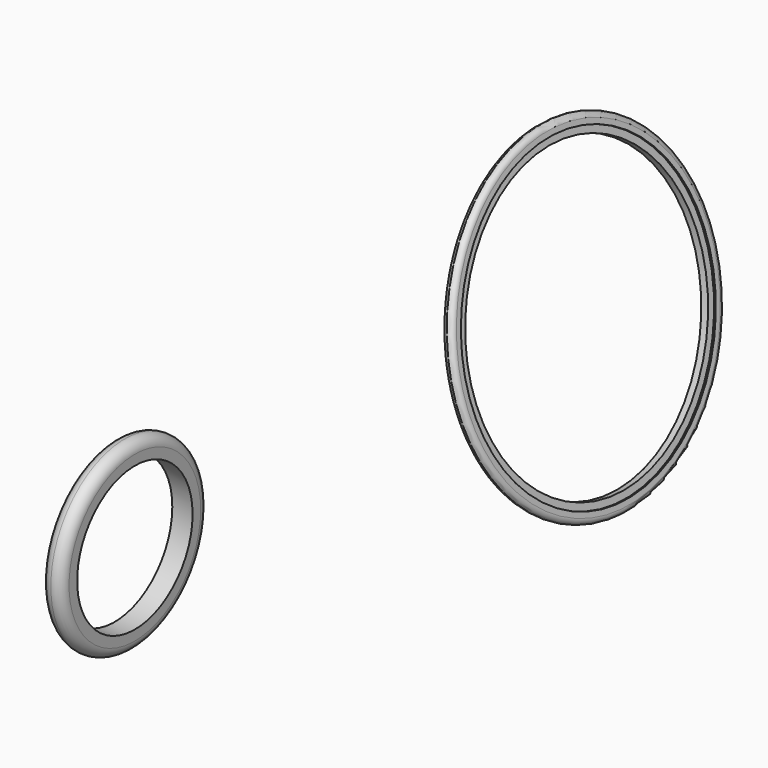
from build123d import *

# Parameters (mm, degrees)
F10_R     = 260.35
F10_R_2   = 203.2
F11_DEPTH = 28.575
F12_R     = 28.57499
F14_R     = 457.2
F14_R_2   = 427.2
F15_DEPTH = 15
F16_R     = 14.99999
F17_R     = 427.2
F17_R_2   = 407.2
F18_DEPTH = 10


# Not quite as in the source:
# - a fillet or chamfer is up to 0.001 mm smaller than in the source, because OpenCascade refuses the exact size


with BuildPart() as f11:
    # F10 (on Right) → F11 (new body, symmetric)
    with BuildSketch(Plane.YZ):
        with Locations((-600, 260.35)):
            Circle(F10_R)
        with Locations((-600, 260.35)):
            Circle(F10_R_2, mode=Mode.SUBTRACT)
    extrude(amount=F11_DEPTH, both=True)

    # F12 (radius 28.575 in the source; OpenCascade refuses exactly that, so slightly less here)
    f12_edges = [f11.edges().sort_by_distance(p)[0] for p in [
        (-28.575, -860.35, 260.35),
        (0, -339.65, 260.35),
        (28.575, -860.35, 260.35),
    ]]
    fillet(f12_edges, radius=F12_R)


with BuildPart() as f15:
    # F14 (on face) → F15 (new body, symmetric)
    with BuildSketch(Plane(origin=(419.8557158515, 0, 112.5), x_dir=(0, 1, 0), z_dir=(0.9659258263, 0, 0.2588190451))):
        with Locations((600, 340.7314297039)):
            Circle(F14_R)
        with Locations((600, 340.7314297039)):
            Circle(F14_R_2, mode=Mode.SUBTRACT)
    extrude(amount=F15_DEPTH, both=True)

    # F16 (radius 15 in the source; OpenCascade refuses exactly that, so slightly less here)
    f16_edges = [f15.edges().sort_by_distance(p)[0] for p in [
        (317.179045, 142.8, 437.739002),
        (331.667933, 1057.2, 441.621288),
        (346.15682, 142.8, 445.503573),
    ]]
    fillet(f16_edges, radius=F16_R)

    # F17 (on face) → F18 (join, symmetric)
    with BuildSketch(Plane(origin=(419.8557158515, 0, 112.5), x_dir=(0, 1, 0), z_dir=(0.9659258263, 0, 0.2588190451))):
        with Locations((600, 340.7314297039)):
            Circle(F17_R)
        with Locations((600, 340.7314297039)):
            Circle(F17_R_2, mode=Mode.SUBTRACT)
    extrude(amount=F18_DEPTH, both=True)


solid = Compound([f11.part, f15.part])
